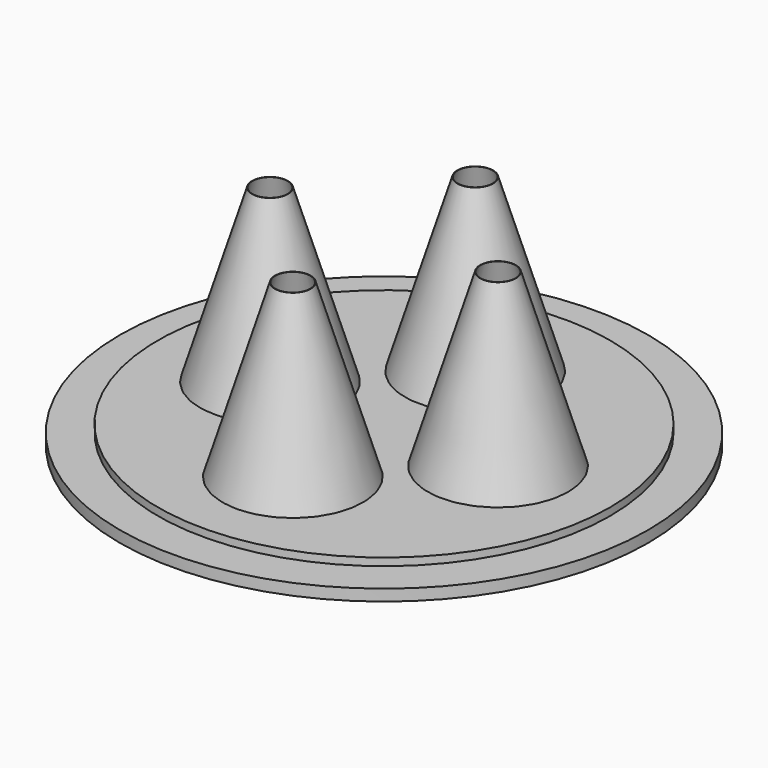
from build123d import *

# Parameters (mm, degrees)
F1_R      = 10
F3_DEPTH  = 25
F3_TAPER  = 17
F2_R      = 29.75
F5_DEPTH  = 2.5
F0_R      = 34.75
F6_DEPTH  = 1.5
F4_R      = 9
F7_DEPTH  = 25.001
F7_TAPER  = 15
F8_COUNT  = 4
F9_R      = 9
F9_R_2    = 8.6463735814
F10_DEPTH = 2.5
F10_TAPER = 17


# Not quite as in the source:
# - a feature names something its author has since deleted; it is built from what else it names


with BuildPart() as f3:
    # F1 (on Top) → F3 (new body)
    with BuildSketch(Plane.XY):
        with Locations((15, 0)):
            Circle(F1_R)
    extrude(amount=F3_DEPTH, taper=F3_TAPER)


with BuildPart() as f5:
    # F2 (on Top) → F5 (new body)
    with BuildSketch(Plane.XY):
        Circle(F2_R)
    extrude(amount=F5_DEPTH)


with BuildPart() as f6:
    # F0 (on Top) → F6 (new body)
    with BuildSketch(Plane.XY):
        Circle(F0_R)
    extrude(amount=F6_DEPTH)


with BuildPart() as f7_tool:
    # F4 (on Top) → F7 (new body, through all)
    with BuildSketch(Plane.XY):
        with Locations((15, 0)):
            Circle(F4_R)
    extrude(amount=F7_DEPTH, taper=F7_TAPER)


with BuildPart() as f3_1:
    add(f3.part)

    # F7: cut by f7_tool
    add(f7_tool.part, mode=Mode.SUBTRACT)


with BuildPart() as f5_1:
    add(f5.part)

    # F7: cut by f7_tool
    add(f7_tool.part, mode=Mode.SUBTRACT)


with BuildPart() as f6_1:
    add(f6.part)

    # F7: cut by f7_tool
    add(f7_tool.part, mode=Mode.SUBTRACT)


with BuildPart() as f8_1:
    # F8: instance of F3
    add(f3_1.part.rotate(Axis((0, 0, 0), (0, 0, 1)), 1 * 360 / F8_COUNT))


with BuildPart() as f8_2:
    # F8: instance of F3
    add(f3_1.part.rotate(Axis((0, 0, 0), (0, 0, 1)), 2 * 360 / F8_COUNT))


with BuildPart() as f8_3:
    # F8: instance of F3
    add(f3_1.part.rotate(Axis((0, 0, 0), (0, 0, 1)), 3 * 360 / F8_COUNT))


with BuildPart() as f10_tool:
    # F9 (on face) → F10 (new body)
    with BuildSketch(Plane.XY.offset(2.5)):
        with Locations((0, -15)):
            Circle(F9_R)
        with Locations((15, 0)):
            Circle(F9_R)
        with Locations((15, 0)):
            Circle(F9_R_2, mode=Mode.SUBTRACT)
        with Locations((0, 15)):
            Circle(F9_R)
        with Locations((-15, 0)):
            Circle(F9_R)
    extrude(amount=-F10_DEPTH, taper=F10_TAPER)


with BuildPart() as f3_2:
    add(f3_1.part)

    # F10: cut by f10_tool
    add(f10_tool.part, mode=Mode.SUBTRACT)


with BuildPart() as f5_2:
    add(f5_1.part)

    # F10: cut by f10_tool
    add(f10_tool.part, mode=Mode.SUBTRACT)


with BuildPart() as f6_2:
    add(f6_1.part)

    # F10: cut by f10_tool
    add(f10_tool.part, mode=Mode.SUBTRACT)


with BuildPart() as f8_1_1:
    add(f8_1.part)

    # F10: cut by f10_tool
    add(f10_tool.part, mode=Mode.SUBTRACT)


with BuildPart() as f8_2_1:
    add(f8_2.part)

    # F10: cut by f10_tool
    add(f10_tool.part, mode=Mode.SUBTRACT)


with BuildPart() as f8_3_1:
    add(f8_3.part)

    # F10: cut by f10_tool
    add(f10_tool.part, mode=Mode.SUBTRACT)


solid = Compound([f3_2.part, f5_2.part, f6_2.part, f8_1_1.part, f8_2_1.part, f8_3_1.part])
